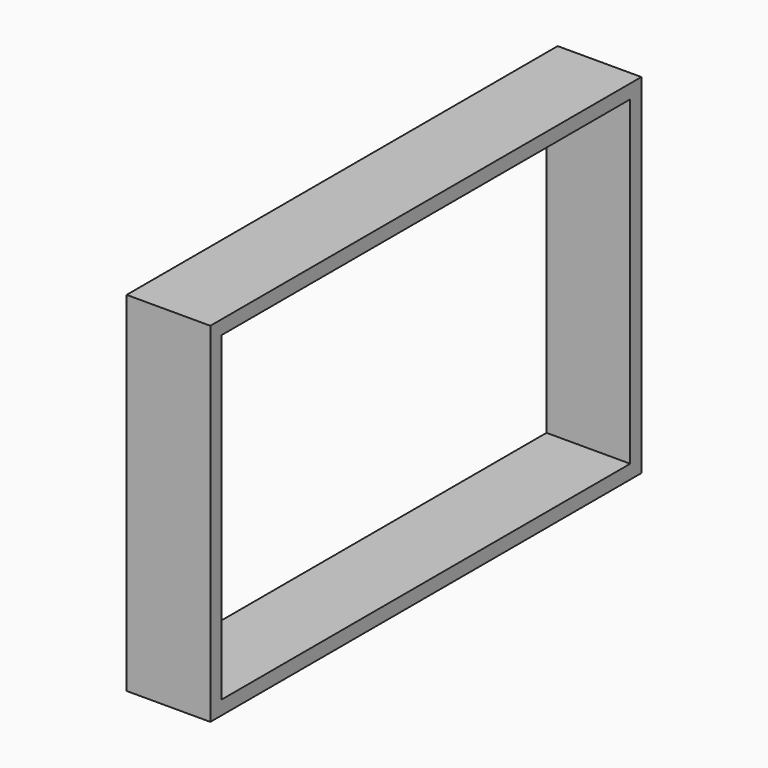
from build123d import *

# Parameters (mm, degrees)
F0_W     = 490.474
F0_H     = 317.5
F0_W_2   = 465.074
F0_H_2   = 292.1
F1_DEPTH = 38.1


# Not quite as in the source:
# - the program builds the solid bodies; features that only make, move or delete a surface that nothing else refers to are left out


with BuildPart() as f1:
    # F0 (on Right) → F1 (new body, symmetric)
    with BuildSketch(Plane.YZ):
        Rectangle(F0_W, F0_H)
        Rectangle(F0_W_2, F0_H_2, mode=Mode.SUBTRACT)
    extrude(amount=F1_DEPTH, both=True)


solid = f1.part
